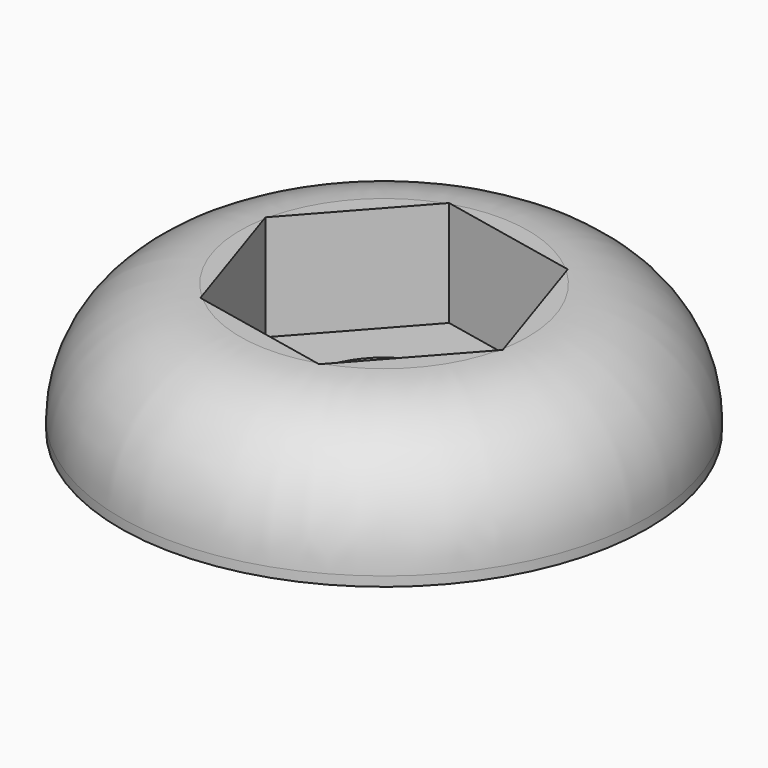
from build123d import *

# Parameters (mm, degrees)
F0_R     = 11
F1_DEPTH = 4.4
F2_R     = 11
F2_R_2   = 3.25
F3_DEPTH = 1


# Not quite as in the source:
# - a fillet or chamfer that OpenCascade refuses, or shapes differently, is made with other operations: its cross-section is extruded or revolved along the edge and cut away or added


with BuildPart() as f1:
    # F0 (on Top) → F1 (new body)
    with BuildSketch(Plane.XY):
        Circle(F0_R)
        Polygon((4.0383603583, 4.521243813), (5.9346921779, -1.2367007534), (1.8963318196, -5.7579445664), (-4.0383603583, -4.521243813), (-5.9346921779, 1.2367007534), (-1.8963318196, 5.7579445664), align=None, mode=Mode.SUBTRACT)
    extrude(amount=F1_DEPTH)

    # F2 (on face) → F3 (join)
    with BuildSketch(Plane(origin=(0, 0, 0), x_dir=(1, 0, 0), z_dir=(0, 0, -1))):
        Circle(F2_R)
        Circle(F2_R_2, mode=Mode.SUBTRACT)
    extrude(amount=F3_DEPTH)

    # F4: fillet of radius 5 on 1 edges, made by hand

    # F4_s1 → F4_t2 (revolve, cut)
    with BuildSketch(Plane.XZ):
        with BuildLine():
            ThreePointArc((11, -0.6), (9.5355339059, 2.9355339059), (6, 4.4))
            Line((6, 4.4), (11, 4.4))
            Line((11, 4.4), (11, -0.6))
        make_face()
    revolve(axis=Axis((0, 0, 4.4), (0, 0, 1)), mode=Mode.SUBTRACT)


solid = f1.part
